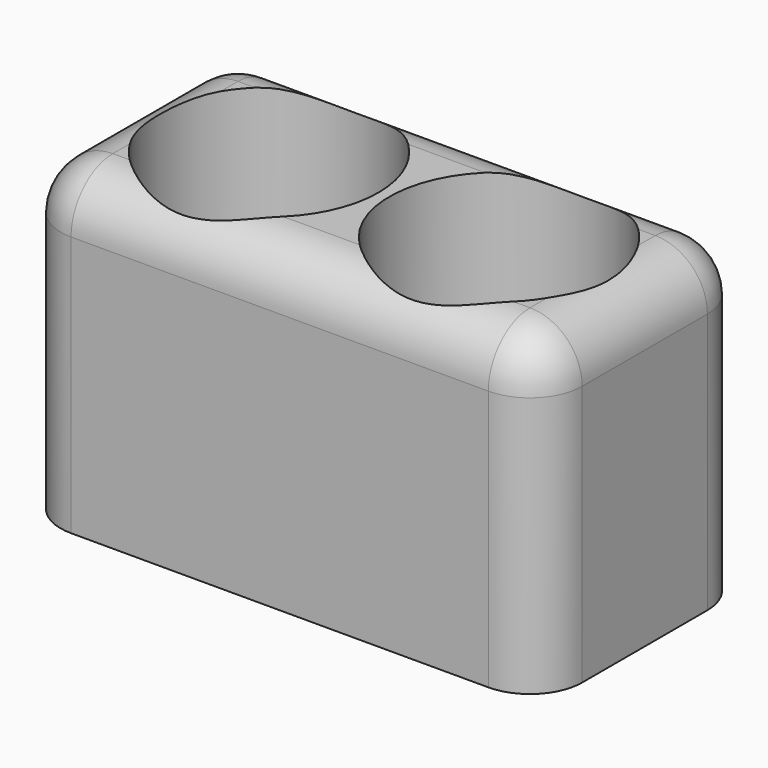
from build123d import *

# Parameters (mm, degrees)
F2_DEPTH     = 30
F3_START     = 5
F0_R         = 10.5
F3_DEPTH     = 55
F4_T1_DEPTH  = 40
F4_T3_DEPTH  = 15
F4_T6_ANGLE  = 90
F4_T8_ANGLE  = 90
F4_T10_ANGLE = 90
F4_T12_ANGLE = 90


# Not quite as in the source:
# - a fillet or chamfer that OpenCascade refuses, or shapes differently, is made with other operations: its cross-section is extruded or revolved along the edge and cut away or added


with BuildPart() as f2:
    # F1 (on Top) → F2 (new body)
    with BuildSketch(Plane.XY):
        with BuildLine():
            Line((31.0264997565, 12.5), (-8.9735002435, 12.5))
            ThreePointArc((-8.9735002435, 12.5), (-12.5090341494, 11.0355339059), (-13.9735002435, 7.5))
            Line((-13.9735002435, 7.5), (-13.9735002435, -7.5))
            ThreePointArc((-13.9735002435, -7.5), (-12.5090341494, -11.0355339059), (-8.9735002435, -12.5))
            Line((-8.9735002435, -12.5), (31.0264997565, -12.5))
            ThreePointArc((31.0264997565, -12.5), (34.5620336625, -11.0355339059), (36.0264997565, -7.5))
            Line((36.0264997565, -7.5), (36.0264997565, 7.5))
            ThreePointArc((36.0264997565, 7.5), (34.5620336625, 11.0355339059), (31.0264997565, 12.5))
        make_face()
    extrude(amount=F2_DEPTH)

    # F0 (on Top) → F3 (cut)
    with BuildSketch(Plane.XY.offset(F3_START)):
        Circle(F0_R)
        with Locations((22.0529995131, 0)):
            Circle(F0_R)
    extrude(amount=F3_DEPTH, mode=Mode.SUBTRACT)

    # F4: fillet of radius 5 on 8 edges, made by hand

    # F4_s2 → F4_t1 (cut)
    with BuildSketch(Plane.YZ.offset(-8.9735002435)):
        with BuildLine():
            ThreePointArc((-7.5, 30), (-11.0355339059, 28.5355339059), (-12.5, 25))
            Line((-12.5, 25), (-12.5, 30))
            Line((-12.5, 30), (-7.5, 30))
        make_face()
        with BuildLine():
            ThreePointArc((12.5, 25), (11.0355339059, 28.5355339059), (7.5, 30))
            Line((7.5, 30), (12.5, 30))
            Line((12.5, 30), (12.5, 25))
        make_face()
    extrude(amount=F4_T1_DEPTH, mode=Mode.SUBTRACT)

    # F4_s4 → F4_t3 (cut)
    with BuildSketch(Plane.XZ.offset(-7.5)):
        with BuildLine():
            ThreePointArc((31.0264997565, 30), (34.5620336625, 28.5355339059), (36.0264997565, 25))
            Line((36.0264997565, 25), (36.0264997565, 30))
            Line((36.0264997565, 30), (31.0264997565, 30))
        make_face()
        with BuildLine():
            ThreePointArc((-8.9735002435, 30), (-12.5090341494, 28.5355339059), (-13.9735002435, 25))
            Line((-13.9735002435, 25), (-13.9735002435, 30))
            Line((-13.9735002435, 30), (-8.9735002435, 30))
        make_face()
    extrude(amount=F4_T3_DEPTH, mode=Mode.SUBTRACT)

    # F4_s5 → F4_t6 (revolve, cut)
    with BuildSketch(Plane.YZ.offset(31.0264997565)):
        with BuildLine():
            ThreePointArc((-7.5, 30), (-11.0355339059, 28.5355339059), (-12.5, 25))
            Line((-12.5, 25), (-12.5, 30))
            Line((-12.5, 30), (-7.5, 30))
        make_face()
    revolve(axis=Axis((31.0264997565, -7.5, 30), (0, 0, 1)), revolution_arc=F4_T6_ANGLE, mode=Mode.SUBTRACT)

    # F4_s7 → F4_t8 (revolve, cut)
    with BuildSketch(Plane.XZ.offset(-7.5)):
        with BuildLine():
            ThreePointArc((36.0264997565, 25), (34.5620336625, 28.5355339059), (31.0264997565, 30))
            Line((31.0264997565, 30), (36.0264997565, 30))
            Line((36.0264997565, 30), (36.0264997565, 25))
        make_face()
    revolve(axis=Axis((31.0264997565, 7.5, 30), (0, 0, 1)), revolution_arc=F4_T8_ANGLE, mode=Mode.SUBTRACT)

    # F4_s9 → F4_t10 (revolve, cut)
    with BuildSketch(Plane.YZ.offset(-8.9735002435)):
        with BuildLine():
            ThreePointArc((12.5, 25), (11.0355339059, 28.5355339059), (7.5, 30))
            Line((7.5, 30), (12.5, 30))
            Line((12.5, 30), (12.5, 25))
        make_face()
    revolve(axis=Axis((-8.9735002435, 7.5, 30), (0, 0, 1)), revolution_arc=F4_T10_ANGLE, mode=Mode.SUBTRACT)

    # F4_s11 → F4_t12 (revolve, cut)
    with BuildSketch(Plane.XZ.offset(7.5)):
        with BuildLine():
            ThreePointArc((-8.9735002435, 30), (-12.5090341494, 28.5355339059), (-13.9735002435, 25))
            Line((-13.9735002435, 25), (-13.9735002435, 30))
            Line((-13.9735002435, 30), (-8.9735002435, 30))
        make_face()
    revolve(axis=Axis((-8.9735002435, -7.5, 30), (0, 0, 1)), revolution_arc=F4_T12_ANGLE, mode=Mode.SUBTRACT)


solid = f2.part
